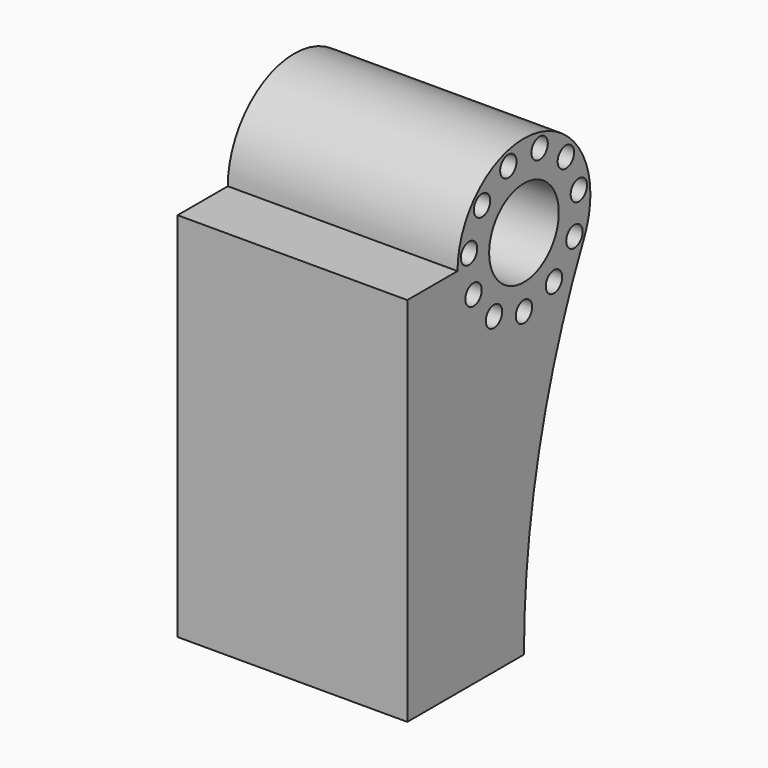
from build123d import *

# Parameters (mm, degrees)
F1_DEPTH = 9.906
F2_DEPTH = 35.56
F4_D     = 6.35
F4_2_D   = 6.35


# Not quite as in the source:
# - a feature of the source that left no trace in its solid (it failed there, or was rolled back) is left out


with BuildPart() as f1:
    # F0 (on Right) → F1 (new body)
    with BuildSketch(Plane.YZ):
        with BuildLine():
            ThreePointArc((45.734231444, 46.3423677323), (36.2491474566, 35.7200728964), (22.5654517973, 31.7759077207))
            Line((22.5654517973, 31.7759077207), (22.5654517973, -57.4847658439))
            ThreePointArc((22.5654517973, -57.4847658439), (28.4280108592, -4.2943860347), (45.734231444, 46.3423677323))
        make_face()
        with BuildLine():
            Line((-3.1434063259, 57.4847658439), (9.0865948156, 57.4847658439))
            ThreePointArc((9.0865948156, 57.4847658439), (22.5654517973, 70.9636228256), (36.044308779, 57.4847658439))
            ThreePointArc((36.044308779, 57.4847658439), (32.0964429717, 47.9537746695), (22.5654517973, 44.0059088622))
            Line((22.5654517973, 44.0059088622), (22.5654517973, 31.7759077207))
            ThreePointArc((22.5654517973, 31.7759077207), (36.2491474566, 35.7200728964), (45.734231444, 46.3423677323))
            ThreePointArc((45.734231444, 46.3423677323), (45.8249787247, 46.5353583121), (45.9158944923, 46.7282695768))
            ThreePointArc((45.9158944923, 46.7282695768), (47.6777854638, 51.9787615014), (48.2743099204, 57.4847658439))
            ThreePointArc((48.2743099204, 57.4847658439), (22.5654517973, 83.193623967), (-3.1434063259, 57.4847658439))
        make_face()
        with BuildLine():
            ThreePointArc((22.5654517973, 44.0059088622), (13.0344606229, 47.9537746695), (9.0865948156, 57.4847658439))
            Line((9.0865948156, 57.4847658439), (-3.1434063259, 57.4847658439))
            ThreePointArc((-3.1434063259, 57.4847658439), (4.3865438818, 39.3058579284), (22.5654517973, 31.7759077207))
            Line((22.5654517973, 31.7759077207), (22.5654517973, 44.0059088622))
        make_face()
        with BuildLine():
            ThreePointArc((22.5654517973, 31.7759077207), (4.3865438818, 39.3058579284), (-3.1434063259, 57.4847658439))
            Line((-3.1434063259, 57.4847658439), (-22.5654517973, 57.4847658439))
            Line((-22.5654517973, 57.4847658439), (-22.5654517973, -57.4847658439))
            Line((-22.5654517973, -57.4847658439), (22.5654517973, -57.4847658439))
            Line((22.5654517973, -57.4847658439), (22.5654517973, 31.7759077207))
        make_face()
    extrude(amount=F1_DEPTH)

    # F4 (through all)
    with Locations(Plane.YZ.offset(35.56)):
        with Locations((38.7895710473, 71.5430452002), (43.8145290766, 60.5399219241), (42.0930552086, 48.5668081792), (22.5654517973, 36.0171794891), (10.9591983617, 39.4250829816), (34.1717052329, 39.4250829816), (3.037848386, 48.5668081792), (1.3163745179, 60.5399219241), (6.3413325473, 71.5430452002), (16.5173338044, 78.0827641117), (28.6135697902, 78.0827641117)):
            Hole(F4_D / 2)


with BuildPart() as f2:
    # F0 (on Right) → F2 (new body, symmetric)
    with BuildSketch(Plane.YZ):
        with BuildLine():
            ThreePointArc((22.5654517973, 44.0059088622), (13.0344606229, 47.9537746695), (9.0865948156, 57.4847658439))
            Line((9.0865948156, 57.4847658439), (-3.1434063259, 57.4847658439))
            ThreePointArc((-3.1434063259, 57.4847658439), (4.3865438818, 39.3058579284), (22.5654517973, 31.7759077207))
            Line((22.5654517973, 31.7759077207), (22.5654517973, 44.0059088622))
        make_face()
        with BuildLine():
            Line((-3.1434063259, 57.4847658439), (9.0865948156, 57.4847658439))
            ThreePointArc((9.0865948156, 57.4847658439), (22.5654517973, 70.9636228256), (36.044308779, 57.4847658439))
            ThreePointArc((36.044308779, 57.4847658439), (32.0964429717, 47.9537746695), (22.5654517973, 44.0059088622))
            Line((22.5654517973, 44.0059088622), (22.5654517973, 31.7759077207))
            ThreePointArc((22.5654517973, 31.7759077207), (36.2491474566, 35.7200728964), (45.734231444, 46.3423677323))
            ThreePointArc((45.734231444, 46.3423677323), (45.8249787247, 46.5353583121), (45.9158944923, 46.7282695768))
            ThreePointArc((45.9158944923, 46.7282695768), (47.6777854638, 51.9787615014), (48.2743099204, 57.4847658439))
            ThreePointArc((48.2743099204, 57.4847658439), (22.5654517973, 83.193623967), (-3.1434063259, 57.4847658439))
        make_face()
        with BuildLine():
            ThreePointArc((22.5654517973, 31.7759077207), (4.3865438818, 39.3058579284), (-3.1434063259, 57.4847658439))
            Line((-3.1434063259, 57.4847658439), (-22.5654517973, 57.4847658439))
            Line((-22.5654517973, 57.4847658439), (-22.5654517973, -57.4847658439))
            Line((-22.5654517973, -57.4847658439), (22.5654517973, -57.4847658439))
            Line((22.5654517973, -57.4847658439), (22.5654517973, 31.7759077207))
        make_face()
        with BuildLine():
            ThreePointArc((45.734231444, 46.3423677323), (36.2491474566, 35.7200728964), (22.5654517973, 31.7759077207))
            Line((22.5654517973, 31.7759077207), (22.5654517973, -57.4847658439))
            ThreePointArc((22.5654517973, -57.4847658439), (28.4280108592, -4.2943860347), (45.734231444, 46.3423677323))
        make_face()
        with BuildLine():
            ThreePointArc((45.9158944923, 46.7282695768), (45.8249787247, 46.5353583121), (45.734231444, 46.3423677323))
            ThreePointArc((45.734231444, 46.3423677323), (45.82586327, 46.5349419129), (45.9158944923, 46.7282695768))
        make_face()
    extrude(amount=F2_DEPTH, both=True)

    # F4#2 (through all)
    with Locations(Plane.YZ.offset(35.56)):
        with Locations((38.7895710473, 71.5430452002), (43.8145290766, 60.5399219241), (42.0930552086, 48.5668081792), (22.5654517973, 36.0171794891), (10.9591983617, 39.4250829816), (34.1717052329, 39.4250829816), (3.037848386, 48.5668081792), (1.3163745179, 60.5399219241), (6.3413325473, 71.5430452002), (16.5173338044, 78.0827641117), (28.6135697902, 78.0827641117)):
            Hole(F4_2_D / 2)


solid = Compound([f1.part, f2.part])
